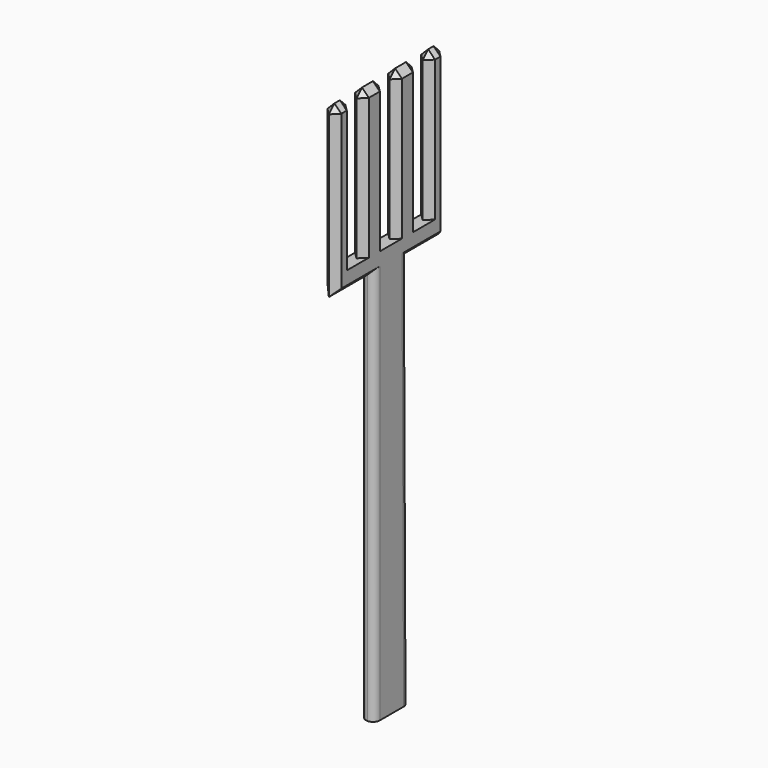
from build123d import *

# Parameters (mm, degrees)
F1_DEPTH = 2.54
F2_R     = 1.26999
F3_SIZE  = 1.26999


# Not quite as in the source:
# - a fillet or chamfer is up to 0.001 mm smaller than in the source, because OpenCascade refuses the exact size


with BuildPart() as f1:
    # F0 (on Right) → F1 (new body)
    with BuildSketch(Plane.YZ):
        Polygon((41.3628902497, -55.5398087384), (48.9828902497, -55.5398087384), (49.3619268672, -55.5398087384), (48.9828902497, 16.8501912616), (57.8728902497, 16.8501912616), (57.8728902497, 20.5470483008), (57.8728902497, 47.7535999747), (54.0628902497, 47.7535999747), (54.0628902497, 20.5470483008), (51.5228902497, 20.5470483008), (51.5228902497, 47.7535999747), (46.4428902497, 47.7535999747), (46.4428902497, 20.5470483008), (43.9028902497, 20.5470483008), (43.9028902497, 47.7535999747), (38.8228902497, 47.7535999747), (38.8228902497, 20.5470483008), (36.2828902497, 20.5470483008), (36.2828902497, 47.7535999747), (32.4728902497, 47.7535999747), (32.4728902497, 16.8502441253), (41.3628902497, 16.8502441253), align=None)
    extrude(amount=F1_DEPTH)

    # F2 (radius 1.27 in the source; OpenCascade refuses exactly that, so slightly less here)
    f2_edges = [f1.edges().sort_by_distance(p)[0] for p in [
        (0, 49.172409, -19.344809),
        (2.54, 41.36289, -19.344782),
        (0, 41.36289, -19.344782),
        (2.54, 49.172409, -19.344809),
    ]]
    fillet(f2_edges, radius=F2_R)

    # F3 (size 1.27 in the source; OpenCascade refuses exactly that, so slightly less here)
    f3_edges = [f1.edges().sort_by_distance(p)[0] for p in [
        (0, 53.42789, 16.850191),
        (2.54, 53.42789, 16.850191),
        (0, 36.91789, 16.850244),
        (2.54, 36.91789, 16.850244),
        (0, 57.87289, 32.301896),
        (2.54, 57.87289, 32.301896),
        (2.54, 54.06289, 34.150324),
        (0, 54.06289, 34.150324),
        (2.54, 36.28289, 34.150324),
        (0, 36.28289, 34.150324),
        (2.54, 43.90289, 34.150324),
        (0, 43.90289, 34.150324),
        (2.54, 51.52289, 34.150324),
        (0, 51.52289, 34.150324),
        (2.54, 32.47289, 32.301922),
        (0, 32.47289, 32.301922),
        (2.54, 38.82289, 34.150324),
        (0, 38.82289, 34.150324),
        (2.54, 46.44289, 34.150324),
        (0, 46.44289, 34.150324),
        (1.27, 51.52289, 47.7536),
        (1.27, 46.44289, 47.7536),
        (0, 48.98289, 47.7536),
        (2.54, 48.98289, 47.7536),
        (1.27, 43.90289, 47.7536),
        (1.27, 38.82289, 47.7536),
        (0, 41.36289, 47.7536),
        (2.54, 41.36289, 47.7536),
        (1.27, 36.28289, 47.7536),
        (1.27, 32.47289, 47.7536),
        (0, 34.37789, 47.7536),
        (2.54, 34.37789, 47.7536),
        (1.27, 57.87289, 47.7536),
        (1.27, 54.06289, 47.7536),
        (0, 55.96789, 47.7536),
        (2.54, 55.96789, 47.7536),
    ]]
    chamfer(f3_edges, length=F3_SIZE)


solid = f1.part
